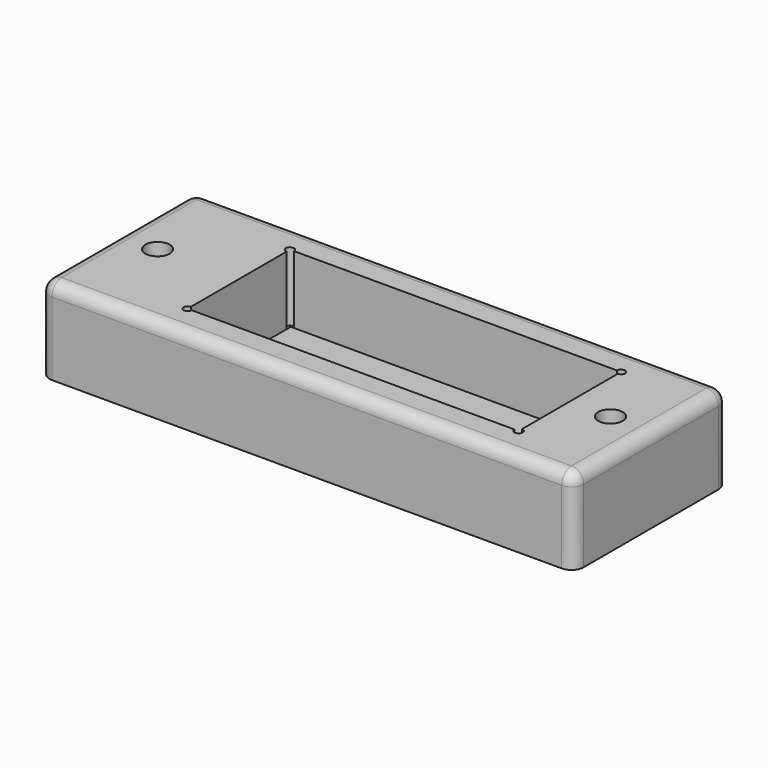
from build123d import *

# Parameters (mm, degrees)
F0_W     = 20
F0_H     = 31.5
F0_R     = 3
F1_DEPTH = 16
F2_DEPTH = 5
F3_W     = 79.5
F3_H     = 29.5
F4_DEPTH = 1
F5_R     = 1
F6_DEPTH = 17
F7_R     = 3


# Not quite as in the source:
# - a feature names something its author has since deleted; it is built from what else it names


with BuildPart() as f1:
    # F0 (on Top) → F1 (new body)
    with BuildSketch(Plane.XY):
        Polygon((-35.75, -15.75), (-35.75, 15.75), (40.25, 15.75), (45.75, 15.75), (65.75, 15.75), (65.75, 23.75), (-65.75, 23.75), (-65.75, -23.75), (65.75, -23.75), (65.75, -15.75), (45.75, -15.75), (20.25, -15.75), align=None)
        Polygon((-51.7662831426, -2.3), (-55.75, -4.6), (-59.7337168574, -2.3), (-59.7337168574, 2.3), (-55.75, 4.6), (-51.7662831426, 2.3), align=None, mode=Mode.SUBTRACT)
        with Locations((55.75, 0)):
            Rectangle(F0_W, F0_H)
        Polygon((59.7337168574, -2.3), (55.75, -4.6), (51.7662831426, -2.3), (51.7662831426, 2.3), (55.75, 4.6), (59.7337168574, 2.3), align=None, mode=Mode.SUBTRACT)
        Polygon((-59.7337168574, -2.3), (-55.75, -4.6), (-51.7662831426, -2.3), (-51.7662831426, 2.3), (-55.75, 4.6), (-59.7337168574, 2.3), align=None)
        with Locations((-55.75, 0)):
            Circle(F0_R, mode=Mode.SUBTRACT)
        Polygon((51.7662831426, -2.3), (55.75, -4.6), (59.7337168574, -2.3), (59.7337168574, 2.3), (55.75, 4.6), (51.7662831426, 2.3), align=None)
        with Locations((55.75, 0)):
            Circle(F0_R, mode=Mode.SUBTRACT)
    extrude(amount=F1_DEPTH)

    # F0 (on Top) → F2 (join)
    with BuildSketch(Plane.XY):
        Polygon((-35.75, -15.75), (-35.75, 15.75), (40.25, 15.75), (45.75, 15.75), (65.75, 15.75), (65.75, 23.75), (-65.75, 23.75), (-65.75, -23.75), (65.75, -23.75), (65.75, -15.75), (45.75, -15.75), (20.25, -15.75), align=None)
        Polygon((-51.7662831426, -2.3), (-55.75, -4.6), (-59.7337168574, -2.3), (-59.7337168574, 2.3), (-55.75, 4.6), (-51.7662831426, 2.3), align=None, mode=Mode.SUBTRACT)
        with Locations((55.75, 0)):
            Rectangle(F0_W, F0_H)
        Polygon((59.7337168574, -2.3), (55.75, -4.6), (51.7662831426, -2.3), (51.7662831426, 2.3), (55.75, 4.6), (59.7337168574, 2.3), align=None, mode=Mode.SUBTRACT)
        Polygon((40.25, 15.75), (-35.75, 15.75), (-35.75, -15.75), (20.25, -15.75), (45.75, -15.75), (45.75, 15.75), align=None)
    extrude(amount=-F2_DEPTH)

    # F3 (on face) → F4 (cut)
    with BuildSketch(Plane.XY):
        Polygon((45.75, 15.75), (40.25, 15.75), (-35.75, 15.75), (-35.75, -15.75), (20.25, -15.75), (45.75, -15.75), align=None)
        with Locations((5, 0)):
            Rectangle(F3_W, F3_H, mode=Mode.SUBTRACT)
    extrude(amount=-F4_DEPTH, mode=Mode.SUBTRACT)

    # F5 (on face) → F6 (cut, through all)
    with BuildSketch(Plane.XY.offset(16)):
        with Locations((45.75, 15.75)):
            Circle(F5_R)
        with Locations((45.75, -15.75)):
            Circle(F5_R)
        with Locations((-35.75, -15.75)):
            Circle(F5_R)
        with Locations((-35.75, 15.75)):
            Circle(F5_R)
    extrude(amount=-F6_DEPTH, mode=Mode.SUBTRACT)

    # F7
    f7_edges = [f1.edges().sort_by_distance(p)[0] for p in [
        (65.75, 23.75, 5.5),
        (65.75, 0, 16),
        (0, 23.75, 16),
        (0, -23.75, 16),
        (65.75, -23.75, 5.5),
        (-65.75, -23.75, 5.5),
        (-65.75, 23.75, 5.5),
        (-65.75, 0, 16),
    ]]
    fillet(f7_edges, radius=F7_R)


solid = f1.part
